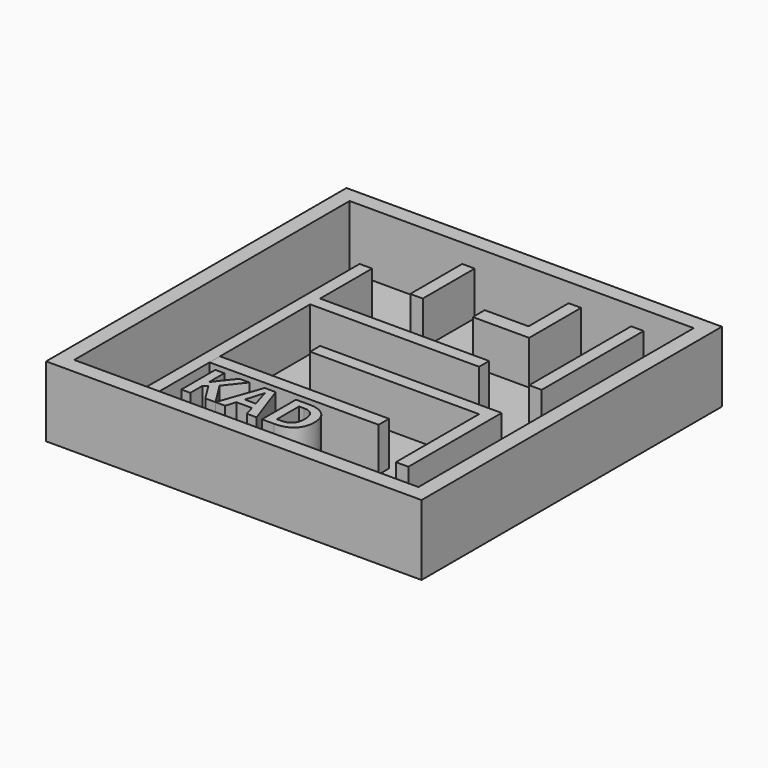
from build123d import *

# Parameters (mm, degrees)
F0_W         = 38.1
F0_H         = 38.1
F1_DEPTH     = 0.79375
F2_W         = 38.1
F2_H         = 38.1
F2_W_2       = 34.925
F2_H_2       = 34.925
F3_DEPTH     = 6.35
F5_DEPTH     = 4.445
F4_W         = 1.27
F4_H         = 6.5922681272
F4_R         = 1.27
F6_DEPTH     = 0.396875
F4_TEXT_SIZE = 6.0444708857
F7_DEPTH     = 4.445
F4_W_2       = 17.145
F4_H_2       = 1.3252556038
F8_DEPTH     = 4.445


# Not quite as in the source:
# - Text() gives the source's letters only with a copy of the font that has no kerning and outlines rounded to 1/6400 em; it was checked with that copy


with BuildPart() as f1:
    # F0 (on Top) → F1 (new body)
    with BuildSketch(Plane.XY):
        with Locations((-7.4162557721, 2.1301306799)):
            Rectangle(F0_W, F0_H)
    extrude(amount=F1_DEPTH)

    # F2 (on face) → F3 (join)
    with BuildSketch(Plane.XY.offset(0.79375)):
        with Locations((-7.4162557721, 2.1301306799)):
            Rectangle(F2_W, F2_H)
        with Locations((-7.4162557721, 2.1301306799)):
            Rectangle(F2_W_2, F2_H_2, mode=Mode.SUBTRACT)
    extrude(amount=F3_DEPTH)

    # F4 (on face) → F6 (cut)
    with BuildSketch(Plane.XY.offset(0.79375)):
        with Locations((7.5062442279, -12.9001028836)):
            Circle(F4_R)
        with Locations((-22.3387557721, -12.4573055655)):
            Circle(F4_R)
    extrude(amount=-F6_DEPTH, mode=Mode.SUBTRACT)


with BuildPart() as f5:
    # F4 (on face) → F5 (new body)
    with BuildSketch(Plane.XY.offset(0.79375)):
        Polygon((-19.7987557721, 14.5126306799), (-19.7987557721, -15.3323693201), (-18.5287557721, -15.3323693201), (-18.5287557721, -6.1048930511), (-18.5287557721, -4.7796374473), (-18.5287557721, 6.6503625527), (-1.3837557721, 6.6503625527), (-1.3837557721, 7.9203625527), (-18.5287557721, 7.9203625527), (-18.5287557721, 14.5126306799), align=None)
    extrude(amount=F5_DEPTH)


with BuildPart() as f5b:
    # F4 (on face) → F5, piece 2 (new body)
    with BuildSketch(Plane.XY.offset(0.79375)):
        with Locations((-12.8137557721, 16.2964966163)):
            Rectangle(F4_W, F4_H)
    extrude(amount=F5_DEPTH)


with BuildPart() as f5c:
    # F4 (on face) → F5, piece 3 (new body)
    with BuildSketch(Plane.XY.offset(0.79375)):
        Polygon((4.9662442279, -10.2523693201), (4.9662442279, 1.5703625527), (-13.4487557721, 1.5703625527), (-13.4487557721, 0.3003625527), (3.6962442279, 0.3003625527), (3.6962442279, -10.2523693201), align=None)
    extrude(amount=F5_DEPTH)


with BuildPart() as f5d:
    # F4 (on face) → F5, piece 4 (new body)
    with BuildSketch(Plane.XY.offset(0.79375)):
        Polygon((4.9662442279, 6.6503625527), (4.9662442279, 19.5926306799), (3.6962442279, 19.5926306799), (3.6962442279, 14.5126306799), (3.6962442279, 13.0003625527), (3.6962442279, 6.6503625527), align=None)
    extrude(amount=F5_DEPTH)


with BuildPart() as f5e:
    # F4 (on face) → F5, piece 5 (new body)
    with BuildSketch(Plane.XY.offset(0.79375)):
        Polygon((-1.3837557721, 19.5926306799), (-2.6537557721, 19.5926306799), (-2.6537557721, 14.5126306799), (-7.0987557721, 14.5126306799), (-7.0987557721, 13.0003625527), (-2.6537557721, 13.0003625527), (-1.3837557721, 13.0003625527), (-1.3837557721, 14.5126306799), align=None)
    extrude(amount=F5_DEPTH)


with BuildPart() as f7:
    # F4 (on face) → F7 (new body)
    with BuildSketch(Plane.XY.offset(0.79375)):
        with Locations((-17.911005998, -11.1428637613)):
            Text('KAD', F4_TEXT_SIZE, font='Open Sans', font_style=FontStyle.BOLD, text_align=(TextAlign.LEFT, TextAlign.BOTTOM))
    extrude(amount=F7_DEPTH)


with BuildPart() as f8:
    # F4 (on face) → F8 (new body)
    with BuildSketch(Plane.XY.offset(0.79375)):
        with Locations((-9.9562557721, -5.4422652492)):
            Rectangle(F4_W_2, F4_H_2)
    extrude(amount=F8_DEPTH)


solid = Compound([f1.part, f5.part, f5b.part, f5c.part, f5d.part, f5e.part, f7.part, f8.part])
